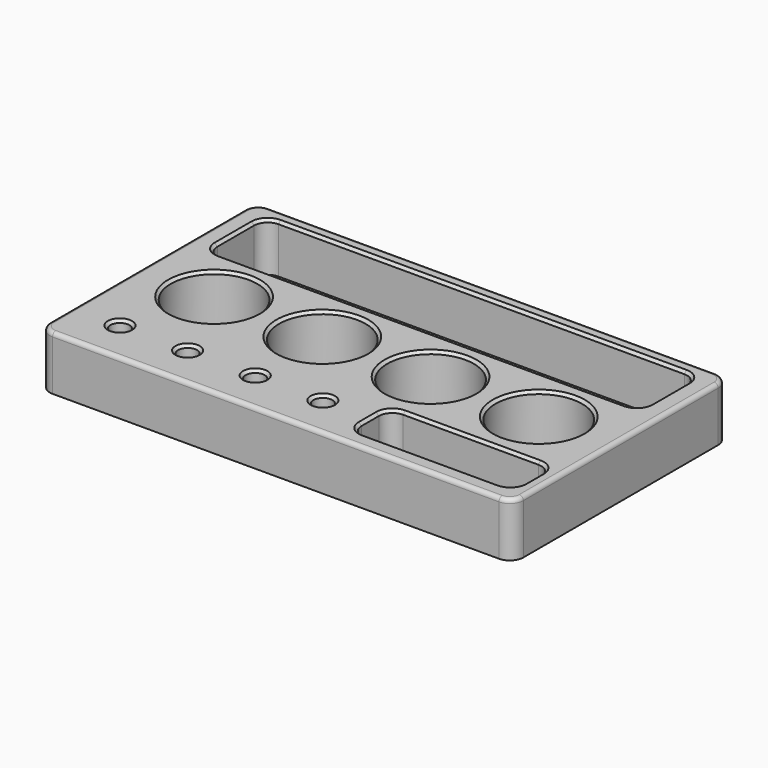
from build123d import *

# Parameters (mm, degrees)
F0_R     = 12.5
F0_R_2   = 18
F0_R_3   = 16
F0_R_4   = 8.5
F0_R_5   = 3.5
F1_DEPTH = 20
F2_DEPTH = 2
F3_R     = 1.5
F4_SIZE  = 1
F5_SIZE  = 1


# Not quite as in the source:
# - a feature names something its author has since deleted; it is built from what else it names


with BuildPart() as f1:
    # F0 (on Top) → F1 (new body)
    with BuildSketch(Plane.XY):
        with BuildLine():
            Line((82.5, 50), (-82.5, 50))
            ThreePointArc((-82.5, 50), (-86.0355339059, 48.5355339059), (-87.5, 45))
            Line((-87.5, 45), (-87.5, -45))
            ThreePointArc((-87.5, -45), (-86.0355339059, -48.5355339059), (-82.5, -50))
            Line((-82.5, -50), (82.5, -50))
            ThreePointArc((82.5, -50), (86.0355339059, -48.5355339059), (87.5, -45))
            Line((87.5, -45), (87.5, 45))
            ThreePointArc((87.5, 45), (86.0355339059, 48.5355339059), (82.5, 50))
        make_face()
        with Locations((-70, -34.5)):
            Circle(F0_R, mode=Mode.SUBTRACT)
        with BuildLine():
            ThreePointArc((-32.5, -34.5), (-45, -47), (-57.5, -34.5))
            ThreePointArc((-57.5, -34.5), (-45, -22), (-32.5, -34.5))
        make_face(mode=Mode.SUBTRACT)
        with BuildLine():
            ThreePointArc((-7.5, -34.5), (-20, -47), (-32.5, -34.5))
            ThreePointArc((-32.5, -34.5), (-20, -22), (-7.5, -34.5))
        make_face(mode=Mode.SUBTRACT)
        with Locations((-60, -3.5)):
            Circle(F0_R_2, mode=Mode.SUBTRACT)
        with Locations((-20, -3.5)):
            Circle(F0_R_2, mode=Mode.SUBTRACT)
        with BuildLine():
            ThreePointArc((17.5, -34.5), (5, -47), (-7.5, -34.5))
            ThreePointArc((-7.5, -34.5), (5, -22), (17.5, -34.5))
        make_face(mode=Mode.SUBTRACT)
        with BuildLine():
            ThreePointArc((20.5, -30.5), (22.5502525317, -25.5502525317), (27.5, -23.5))
            Line((27.5, -23.5), (77.5, -23.5))
            ThreePointArc((77.5, -23.5), (82.4497474683, -25.5502525317), (84.5, -30.5))
            Line((84.5, -30.5), (84.5, -38.5))
            ThreePointArc((84.5, -38.5), (82.4497474683, -43.4497474683), (77.5, -45.5))
            Line((77.5, -45.5), (27.5, -45.5))
            ThreePointArc((27.5, -45.5), (22.5502525317, -43.4497474683), (20.5, -38.5))
            Line((20.5, -38.5), (20.5, -30.5))
        make_face(mode=Mode.SUBTRACT)
        with Locations((20, -3.5)):
            Circle(F0_R_2, mode=Mode.SUBTRACT)
        with Locations((60, -3.5)):
            Circle(F0_R_2, mode=Mode.SUBTRACT)
        with BuildLine():
            ThreePointArc((82, 23), (79.9497474683, 18.0502525317), (75, 16))
            Line((75, 16), (-75, 16))
            ThreePointArc((-75, 16), (-79.9497474683, 18.0502525317), (-82, 23))
            Line((-82, 23), (-82, 40))
            ThreePointArc((-82, 40), (-79.9497474683, 44.9497474683), (-75, 47))
            Line((-75, 47), (75, 47))
            ThreePointArc((75, 47), (79.9497474683, 44.9497474683), (82, 40))
            Line((82, 40), (82, 23))
        make_face(mode=Mode.SUBTRACT)
        with BuildLine():
            Line((-75, 16), (75, 16))
            ThreePointArc((75, 16), (79.9497474683, 18.0502525317), (82, 23))
            Line((82, 23), (82, 40))
            ThreePointArc((82, 40), (79.9497474683, 44.9497474683), (75, 47))
            Line((75, 47), (-75, 47))
            ThreePointArc((-75, 47), (-79.9497474683, 44.9497474683), (-82, 40))
            Line((-82, 40), (-82, 23))
            ThreePointArc((-82, 23), (-79.9497474683, 18.0502525317), (-75, 16))
        make_face()
        with BuildLine():
            ThreePointArc((80, 23), (78.5355339059, 19.4644660941), (75, 18))
            Line((75, 18), (-75, 18))
            ThreePointArc((-75, 18), (-78.5355339059, 19.4644660941), (-80, 23))
            Line((-80, 23), (-80, 40))
            ThreePointArc((-80, 40), (-78.5355339059, 43.5355339059), (-75, 45))
            Line((-75, 45), (75, 45))
            ThreePointArc((75, 45), (78.5355339059, 43.5355339059), (80, 40))
            Line((80, 40), (80, 23))
        make_face(mode=Mode.SUBTRACT)
        with Locations((60, -3.5)):
            Circle(F0_R_2)
        with Locations((60, -3.5)):
            Circle(F0_R_3, mode=Mode.SUBTRACT)
        with Locations((20, -3.5)):
            Circle(F0_R_2)
        with Locations((20, -3.5)):
            Circle(F0_R_3, mode=Mode.SUBTRACT)
        with Locations((-20, -3.5)):
            Circle(F0_R_2)
        with Locations((-20, -3.5)):
            Circle(F0_R_3, mode=Mode.SUBTRACT)
        with Locations((-60, -3.5)):
            Circle(F0_R_2)
        with Locations((-60, -3.5)):
            Circle(F0_R_3, mode=Mode.SUBTRACT)
        with Locations((-70, -34.5)):
            Circle(F0_R)
        with Locations((-70, -34.5)):
            Circle(F0_R_4, mode=Mode.SUBTRACT)
        with Locations((-70, -34.5)):
            Circle(F0_R_4)
        with Locations((-70, -34.5)):
            Circle(F0_R_5, mode=Mode.SUBTRACT)
        with BuildLine():
            ThreePointArc((-32.5, -34.5), (-45, -22), (-57.5, -34.5))
            ThreePointArc((-57.5, -34.5), (-45, -47), (-32.5, -34.5))
        make_face()
        with Locations((-45, -34.5)):
            Circle(F0_R_4, mode=Mode.SUBTRACT)
        with Locations((-45, -34.5)):
            Circle(F0_R_4)
        with Locations((-45, -34.5)):
            Circle(F0_R_5, mode=Mode.SUBTRACT)
        with BuildLine():
            ThreePointArc((-7.5, -34.5), (-20, -22), (-32.5, -34.5))
            ThreePointArc((-32.5, -34.5), (-20, -47), (-7.5, -34.5))
        make_face()
        with Locations((-20, -34.5)):
            Circle(F0_R_4, mode=Mode.SUBTRACT)
        with Locations((-20, -34.5)):
            Circle(F0_R_4)
        with Locations((-20, -34.5)):
            Circle(F0_R_5, mode=Mode.SUBTRACT)
        with BuildLine():
            ThreePointArc((17.5, -34.5), (5, -22), (-7.5, -34.5))
            ThreePointArc((-7.5, -34.5), (5, -47), (17.5, -34.5))
        make_face()
        with Locations((5, -34.5)):
            Circle(F0_R_4, mode=Mode.SUBTRACT)
        with Locations((5, -34.5)):
            Circle(F0_R_4)
        with Locations((5, -34.5)):
            Circle(F0_R_5, mode=Mode.SUBTRACT)
        with BuildLine():
            Line((77.5, -23.5), (27.5, -23.5))
            ThreePointArc((27.5, -23.5), (22.5502525317, -25.5502525317), (20.5, -30.5))
            Line((20.5, -30.5), (20.5, -38.5))
            ThreePointArc((20.5, -38.5), (22.5502525317, -43.4497474683), (27.5, -45.5))
            Line((27.5, -45.5), (77.5, -45.5))
            ThreePointArc((77.5, -45.5), (82.4497474683, -43.4497474683), (84.5, -38.5))
            Line((84.5, -38.5), (84.5, -30.5))
            ThreePointArc((84.5, -30.5), (82.4497474683, -25.5502525317), (77.5, -23.5))
        make_face()
        with BuildLine():
            Line((27.5, -25.5), (77.5, -25.5))
            ThreePointArc((77.5, -25.5), (81.0355339059, -26.9644660941), (82.5, -30.5))
            Line((82.5, -30.5), (82.5, -38.5))
            ThreePointArc((82.5, -38.5), (81.0355339059, -42.0355339059), (77.5, -43.5))
            Line((77.5, -43.5), (27.5, -43.5))
            ThreePointArc((27.5, -43.5), (23.9644660941, -42.0355339059), (22.5, -38.5))
            Line((22.5, -38.5), (22.5, -30.5))
            ThreePointArc((22.5, -30.5), (23.9644660941, -26.9644660941), (27.5, -25.5))
        make_face(mode=Mode.SUBTRACT)
    extrude(amount=F1_DEPTH)

    # F0 (on Top) → F2 (join)
    with BuildSketch(Plane.XY):
        with Locations((-60, -3.5)):
            Circle(F0_R_3)
        with Locations((-20, -3.5)):
            Circle(F0_R_3)
        with Locations((60, -3.5)):
            Circle(F0_R_3)
        with BuildLine():
            Line((-75, 18), (75, 18))
            ThreePointArc((75, 18), (78.5355339059, 19.4644660941), (80, 23))
            Line((80, 23), (80, 40))
            ThreePointArc((80, 40), (78.5355339059, 43.5355339059), (75, 45))
            Line((75, 45), (-75, 45))
            ThreePointArc((-75, 45), (-78.5355339059, 43.5355339059), (-80, 40))
            Line((-80, 40), (-80, 23))
            ThreePointArc((-80, 23), (-78.5355339059, 19.4644660941), (-75, 18))
        make_face()
        with BuildLine():
            ThreePointArc((82.5, -30.5), (81.0355339059, -26.9644660941), (77.5, -25.5))
            Line((77.5, -25.5), (27.5, -25.5))
            ThreePointArc((27.5, -25.5), (23.9644660941, -26.9644660941), (22.5, -30.5))
            Line((22.5, -30.5), (22.5, -38.5))
            ThreePointArc((22.5, -38.5), (23.9644660941, -42.0355339059), (27.5, -43.5))
            Line((27.5, -43.5), (77.5, -43.5))
            ThreePointArc((77.5, -43.5), (81.0355339059, -42.0355339059), (82.5, -38.5))
            Line((82.5, -38.5), (82.5, -30.5))
        make_face()
        with Locations((20, -3.5)):
            Circle(F0_R_3)
    extrude(amount=F2_DEPTH)

    # F3
    f3_edges = [f1.edges().sort_by_distance(p)[0] for p in [
        (0, -50, 20),
    ]]
    fillet(f3_edges, radius=F3_R)

    # F4
    f4_edges = [f1.edges().sort_by_distance(p)[0] for p in [
        (-76, -3.5, 20),
        (-36, -3.5, 20),
        (44, -3.5, 20),
        (-78.535534, 43.535534, 20),
        (-80, 31.5, 20),
        (22.5, -30.5, 11),
        (23.964466, -26.964466, 20),
        (4, -3.5, 20),
    ]]
    chamfer(f4_edges, length=F4_SIZE)

    # F5
    f5_edges = [f1.edges().sort_by_distance(p)[0] for p in [
        (-73.5, -34.5, 20),
        (-48.5, -34.5, 20),
        (-23.5, -34.5, 20),
        (1.5, -34.5, 20),
    ]]
    chamfer(f5_edges, length=F5_SIZE)


solid = f1.part
